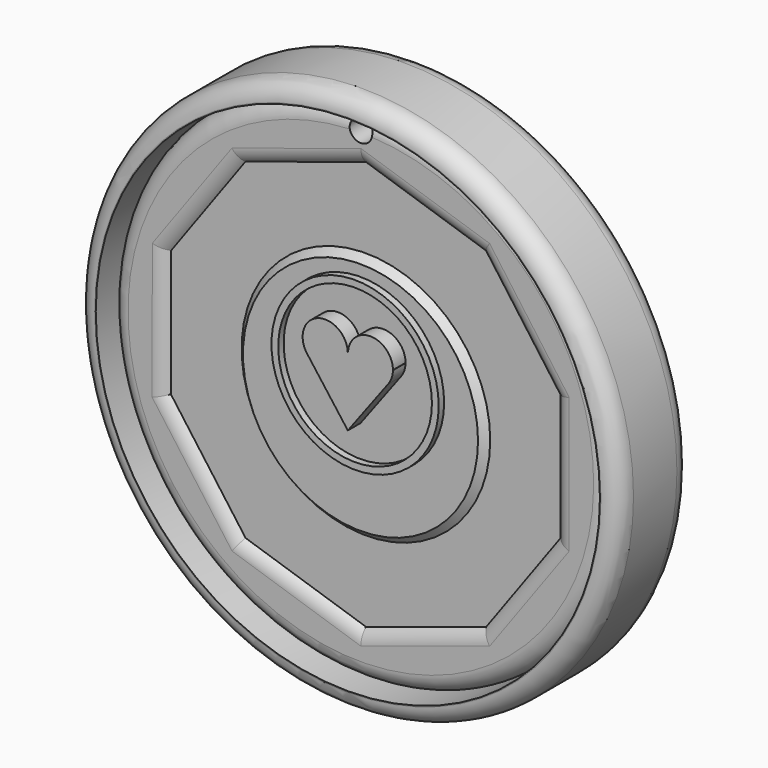
from build123d import *

# Parameters (mm, degrees)
F0_R          = 76.2
F0_R_2        = 70.8290546177
F1_DEPTH      = 25.4
F2_R          = 5.08
F4_DEPTH      = 20.828
F5_R          = 58.42
F6_DEPTH      = 19.05
F7_R          = 38.1
F8_DEPTH      = 20.955
F9_T4_DEPTH   = 54.8412301486
F9_T10_DEPTH  = 54.8210989977
F9_T16_DEPTH  = 54.8418216268
F9_T22_DEPTH  = 54.834061941
F9_T28_DEPTH  = 54.8364529893
F9_T34_DEPTH  = 54.8922066352
F9_T40_DEPTH  = 54.8735006381
F9_T46_DEPTH  = 54.8412936205
F9_T52_DEPTH  = 54.8773174101
F9_T58_DEPTH  = 54.8413615597
F9_T67_DEPTH  = 54.8412301486
F9_T71_DEPTH  = 54.8413615597
F9_T78_DEPTH  = 54.8412301486
F9_T82_DEPTH  = 54.8210989977
F9_T89_DEPTH  = 54.8210989977
F9_T93_DEPTH  = 54.8418216268
F9_T100_DEPTH = 54.8418216268
F9_T104_DEPTH = 54.834061941
F9_T111_DEPTH = 54.834061941
F9_T115_DEPTH = 54.8364529893
F9_T122_DEPTH = 54.8364529893
F9_T126_DEPTH = 54.8922066352
F9_T133_DEPTH = 54.8922066352
F9_T137_DEPTH = 54.8735006381
F9_T144_DEPTH = 54.8735006381
F9_T148_DEPTH = 54.8412936205
F9_T155_DEPTH = 54.8412936205
F9_T159_DEPTH = 54.8773174101
F9_T166_DEPTH = 54.8773174101
F9_T170_DEPTH = 54.8413615597
F12_DEPTH     = 25.4
F14_D         = 6.35
F15_R         = 23.495
F15_R_2       = 21.59
F16_DEPTH     = 22.86


# Not quite as in the source:
# - a fillet or chamfer that OpenCascade refuses, or shapes differently, is made with other operations: its cross-section is extruded or revolved along the edge and cut away or added
# - a feature names something its author has since deleted; it is built from what else it names


with BuildPart() as f1:
    # F0 (on Front) → F1 (new body)
    with BuildSketch(Plane.XZ):
        Circle(F0_R)
        Circle(F0_R_2, mode=Mode.SUBTRACT)
    extrude(amount=F1_DEPTH)

    # F2
    f2_edges = [f1.edges().sort_by_distance(p)[0] for p in [
        (76.2, -12.7, 0),
        (-76.2, 0, 0),
        (-76.2, -25.4, 0),
    ]]
    fillet(f2_edges, radius=F2_R)


with BuildPart() as f4:
    # F3 (on Front) → F4 (new body)
    with BuildSketch(Plane.XZ):
        with BuildLine():
            ThreePointArc((66.9302043248, -22.1240943887), (69.5958852645, -11.2044882855), (70.4920407102, 0))
            ThreePointArc((70.4920407102, 0), (69.6666544261, 10.7556991663), (67.2098243524, 21.2595229017))
            Line((67.2098243524, 21.2595229017), (54.6848949384, 17.7593848735))
            Line((54.6848949384, 17.7593848735), (54.6797294814, -17.7593848735))
            Line((54.6797294814, -17.7593848735), (66.9302043248, -22.1240943887))
        make_face()
        with BuildLine():
            Line((54.6848949384, 17.7593848735), (67.2098243524, 21.2595229017))
            ThreePointArc((67.2098243524, 21.2595229017), (57.3909347279, 40.9317531329), (41.9889338997, 56.6220560687))
            Line((41.9889338997, 56.6220560687), (33.8033564444, 46.5165553507))
            Line((33.8033564444, 46.5165553507), (54.6848949384, 17.7593848735))
        make_face()
        with BuildLine():
            ThreePointArc((41.8571007117, -56.719581482), (57.0778535518, -41.3672145231), (66.9302043248, -22.1240943887))
            Line((66.9302043248, -22.1240943887), (54.6797294814, -17.7593848735))
            Line((54.6797294814, -17.7593848735), (33.7952184523, -46.5151276761))
            Line((33.7952184523, -46.5151276761), (41.8571007117, -56.719581482))
        make_face()
        with BuildLine():
            Line((33.8033564444, 46.5165553507), (41.9889338997, 56.6220560687))
            ThreePointArc((41.9889338997, 56.6220560687), (22.1102184747, 66.9347894781), (0, 70.4920407102))
            Line((0, 70.4920407102), (0, 57.4872407102))
            Line((0, 57.4872407102), (33.8033564444, 46.5165553507))
        make_face()
        with BuildLine():
            ThreePointArc((0, -70.4920407102), (22.0323484517, -66.960461656), (41.8571007117, -56.719581482))
            Line((41.8571007117, -56.719581482), (33.7952184523, -46.5151276761))
            Line((33.7952184523, -46.5151276761), (0, -57.4872407102))
            Line((0, -57.4872407102), (0, -70.4920407102))
        make_face()
        with BuildLine():
            Line((0, 57.4872407102), (0, 70.4920407102))
            ThreePointArc((0, 70.4920407102), (-22.5082471688, 66.8019955755), (-42.6600170071, 56.1181855768))
            Line((-42.6600170071, 56.1181855768), (-33.8520696606, 46.5502763705))
            Line((-33.8520696606, 46.5502763705), (0, 57.4872407102))
        make_face()
        with BuildLine():
            ThreePointArc((-40.8179057709, -57.4719616158), (-21.422090766, -67.1581851355), (0, -70.4920407102))
            Line((0, -70.4920407102), (0, -57.4872407102))
            Line((0, -57.4872407102), (-33.8003104429, -46.5230722268))
            Line((-33.8003104429, -46.5230722268), (-40.8179057709, -57.4719616158))
        make_face()
        with BuildLine():
            Line((-33.8520696606, 46.5502763705), (-42.6600170071, 56.1181855768))
            ThreePointArc((-42.6600170071, 56.1181855768), (-57.0935427408, 41.3455581748), (-66.6260754104, 23.0237676955))
            Line((-66.6260754104, 23.0237676955), (-54.722988429, 17.7853191319))
            Line((-54.722988429, 17.7853191319), (-33.8520696606, 46.5502763705))
        make_face()
        with BuildLine():
            ThreePointArc((-67.6308946717, -19.8793835265), (-57.3897731413, -40.9333817596), (-40.8179057709, -57.4719616158))
            Line((-40.8179057709, -57.4719616158), (-33.8003104429, -46.5230722268))
            Line((-33.8003104429, -46.5230722268), (-54.7957226795, -17.7857782694))
            Line((-54.7957226795, -17.7857782694), (-67.6308946717, -19.8793835265))
        make_face()
        with BuildLine():
            Line((-54.722988429, 17.7853191319), (-66.6260754104, 23.0237676955))
            ThreePointArc((-66.6260754104, 23.0237676955), (-70.4727152882, 1.6505160973), (-67.6308946717, -19.8793835265))
            Line((-67.6308946717, -19.8793835265), (-54.7957226795, -17.7857782694))
            Line((-54.7957226795, -17.7857782694), (-54.722988429, 17.7853191319))
        make_face()
    extrude(amount=F4_DEPTH)

    # F5 (on Front) → F6 (join)
    with BuildSketch(Plane.XZ):
        Circle(F5_R)
    extrude(amount=F6_DEPTH)

    # F7 (on Front) → F8 (join)
    with BuildSketch(Plane.XZ):
        Circle(F7_R)
    extrude(amount=F8_DEPTH)

    # F9: fillet of radius 5.08 on 11 edges, made by hand


with BuildPart() as f9_tool2:
    # F9_s3 → F9_t4 (new body)
    with BuildSketch(Plane(origin=(-16.1166422443, 0, 22.1951571561), x_dir=(0, 1, 0), z_dir=(0.5875684882, 0, -0.8091744383))):
        with BuildLine():
            ThreePointArc((-20.828, 58.5449398441), (-20.3621391396, 56.4198233767), (-19.05, 54.6844740691))
            Line((-19.05, 54.6844740691), (-20.828, 54.6844740691))
            Line((-20.828, 54.6844740691), (-20.828, 58.5449398441))
        make_face()
    extrude(amount=F9_T4_DEPTH)

    split(bisect_by=Plane(origin=(54.6823110534, 0, -0.0079523905), x_dir=(0, 1, 0), z_dir=(-0.9999999894, 0, 0.0001454289)), keep=Keep.TOP)

    split(bisect_by=Plane(origin=(16.8792770905, 0, 52.0091681892), x_dir=(0, 1, 0), z_dir=(-0.3086939776, 0, -0.9511614102)), keep=Keep.TOP)


with BuildPart() as f4_1:
    add(f4.part)

    # F9_t1: cut F9_tool2
    add(f9_tool2.part, mode=Mode.SUBTRACT)


with BuildPart() as f9_tool8:
    # F9_s9 → F9_t10 (new body)
    with BuildSketch(Plane(origin=(0.0039874436, 0, 27.4185015995), x_dir=(0, 1, 0), z_dir=(-0.0001454289, 0, -0.9999999894))):
        with BuildLine():
            ThreePointArc((-20.828, 58.5427774067), (-20.3621391396, 56.4176609393), (-19.05, 54.6823116317))
            Line((-19.05, 54.6823116317), (-20.828, 54.6823116317))
            Line((-20.828, 54.6823116317), (-20.828, 58.5427774067))
        make_face()
    extrude(amount=F9_T10_DEPTH)

    split(bisect_by=Plane(origin=(44.2492785906, 0, 32.1308737575), x_dir=(0, 1, 0), z_dir=(-0.8091744383, 0, -0.5875684882)), keep=Keep.TOP)

    split(bisect_by=Plane(origin=(44.2416517248, 0, -32.1315039481), x_dir=(0, 1, 0), z_dir=(-0.8091207999, 0, 0.5876423497)), keep=Keep.TOP)


with BuildPart() as f4_2:
    add(f4_1.part)

    # F9_t7: cut F9_tool8
    add(f9_tool8.part, mode=Mode.SUBTRACT)


with BuildPart() as f9_tool14:
    # F9_s15 → F9_t16 (new body)
    with BuildSketch(Plane(origin=(16.1095107044, 0, 22.181076964), x_dir=(0, 1, 0), z_dir=(-0.5876423497, 0, -0.8091207999))):
        with BuildLine():
            ThreePointArc((-20.828, 58.5391388871), (-20.3621391396, 56.4140224197), (-19.05, 54.6786731121))
            Line((-19.05, 54.6786731121), (-20.828, 54.6786731121))
            Line((-20.828, 54.6786731121), (-20.828, 58.5391388871))
        make_face()
    extrude(amount=F9_T16_DEPTH)

    split(bisect_by=Plane(origin=(54.6823110534, 0, -0.0079523905), x_dir=(0, 1, 0), z_dir=(-0.9999999894, 0, 0.0001454289)), keep=Keep.TOP)

    split(bisect_by=Plane(origin=(16.8843448329, 0, -52.0054906728), x_dir=(0, 1, 0), z_dir=(-0.3087975758, 0, 0.9511277817)), keep=Keep.TOP)


with BuildPart() as f4_3:
    add(f4_2.part)

    # F9_t13: cut F9_tool14
    add(f9_tool14.part, mode=Mode.SUBTRACT)


with BuildPart() as f9_tool20:
    # F9_s21 → F9_t22 (new body)
    with BuildSketch(Plane(origin=(26.0903642421, 0, 8.4706191785), x_dir=(0, 1, 0), z_dir=(-0.9511277817, 0, -0.3087975758))):
        with BuildLine():
            ThreePointArc((-20.828, 58.5381775099), (-20.3621391396, 56.4130610425), (-19.05, 54.6777117348))
            Line((-19.05, 54.6777117348), (-20.828, 54.6777117348))
            Line((-20.828, 54.6777117348), (-20.828, 58.5381775099))
        make_face()
    extrude(amount=F9_T22_DEPTH)

    split(bisect_by=Plane(origin=(44.2416517248, 0, -32.1315039481), x_dir=(0, 1, 0), z_dir=(-0.8091207999, 0, 0.5876423497)), keep=Keep.TOP)

    split(bisect_by=Plane(origin=(-16.8723907072, 0, -52.0141627411), x_dir=(0, 1, 0), z_dir=(0.3085532219, 0, 0.9512070801)), keep=Keep.TOP)


with BuildPart() as f4_4:
    add(f4_3.part)

    # F9_t19: cut F9_tool20
    add(f9_tool20.part, mode=Mode.SUBTRACT)


with BuildPart() as f9_tool26:
    # F9_s27 → F9_t28 (new body)
    with BuildSketch(Plane(origin=(26.0526466514, 0, -8.4509758515), x_dir=(0, 1, 0), z_dir=(-0.9512070801, 0, 0.3085532219))):
        with BuildLine():
            ThreePointArc((-20.828, 58.5427361543), (-20.3621391396, 56.4176196869), (-19.05, 54.6822703793))
            Line((-19.05, 54.6822703793), (-20.828, 54.6822703793))
            Line((-20.828, 54.6822703793), (-20.828, 58.5427361543))
        make_face()
    extrude(amount=F9_T28_DEPTH)

    split(bisect_by=Plane(origin=(16.8843448329, 0, -52.0054906728), x_dir=(0, 1, 0), z_dir=(-0.3087975758, 0, 0.9511277817)), keep=Keep.TOP)

    split(bisect_by=Plane(origin=(-44.1981655034, 0, -32.2910955438), x_dir=(0, 1, 0), z_dir=(0.8074569447, 0, 0.589926506)), keep=Keep.TOP)


with BuildPart() as f4_5:
    add(f4_4.part)

    # F9_t25: cut F9_tool26
    add(f9_tool26.part, mode=Mode.SUBTRACT)


with BuildPart() as f9_tool32:
    # F9_s33 → F9_t34 (new body)
    with BuildSketch(Plane(origin=(16.0913327762, 0, -22.0248764322), x_dir=(0, 1, 0), z_dir=(-0.589926506, 0, 0.8074569447))):
        with BuildLine():
            ThreePointArc((-20.828, 58.5979546221), (-20.3621391396, 56.4728381547), (-19.05, 54.7374888471))
            Line((-19.05, 54.7374888471), (-20.828, 54.7374888471))
            Line((-20.828, 54.7374888471), (-20.828, 58.5979546221))
        make_face()
    extrude(amount=F9_T34_DEPTH)

    split(bisect_by=Plane(origin=(-16.8723907072, 0, -52.0141627411), x_dir=(0, 1, 0), z_dir=(0.3085532219, 0, 0.9512070801)), keep=Keep.TOP)

    split(bisect_by=Plane(origin=(-54.7591261352, 0, 0.1119691067), x_dir=(0, 1, 0), z_dir=(0.9999979095, 0, -0.0020447527)), keep=Keep.TOP)


with BuildPart() as f4_6:
    add(f4_5.part)

    # F9_t31: cut F9_tool32
    add(f9_tool32.part, mode=Mode.SUBTRACT)


with BuildPart() as f9_tool38:
    # F9_s39 → F9_t40 (new body)
    with BuildSketch(Plane(origin=(-0.0563307891, 0, -27.5488916378), x_dir=(0, 1, 0), z_dir=(0.0020447527, 0, 0.9999979095))):
        with BuildLine():
            ThreePointArc((-20.828, 58.6197063849), (-20.3621391396, 56.4945899175), (-19.05, 54.7592406099))
            Line((-19.05, 54.7592406099), (-20.828, 54.7592406099))
            Line((-20.828, 54.7592406099), (-20.828, 58.6197063849))
        make_face()
    extrude(amount=F9_T40_DEPTH)

    split(bisect_by=Plane(origin=(-44.1981655034, 0, -32.2910955438), x_dir=(0, 1, 0), z_dir=(0.8074569447, 0, 0.589926506)), keep=Keep.TOP)

    split(bisect_by=Plane(origin=(-44.3037877316, 0, 32.1453895171), x_dir=(0, 1, 0), z_dir=(0.8093920981, 0, -0.5872686196)), keep=Keep.TOP)


with BuildPart() as f4_7:
    add(f4_6.part)

    # F9_t37: cut F9_tool38
    add(f9_tool38.part, mode=Mode.SUBTRACT)


with BuildPart() as f9_tool44:
    # F9_s45 → F9_t46 (new body)
    with BuildSketch(Plane(origin=(-16.0870267142, 0, -22.1716466182), x_dir=(0, 1, 0), z_dir=(0.5872686196, 0, 0.8093920981))):
        with BuildLine():
            ThreePointArc((-20.828, 58.5975800082), (-20.3621391396, 56.4724635408), (-19.05, 54.7371142332))
            Line((-19.05, 54.7371142332), (-20.828, 54.7371142332))
            Line((-20.828, 54.7371142332), (-20.828, 58.5975800082))
        make_face()
    extrude(amount=F9_T46_DEPTH)

    split(bisect_by=Plane(origin=(-54.7591261352, 0, 0.1119691067), x_dir=(0, 1, 0), z_dir=(0.9999979095, 0, -0.0020447527)), keep=Keep.TOP)

    split(bisect_by=Plane(origin=(-16.8175972659, 0, 52.0537926693), x_dir=(0, 1, 0), z_dir=(0.3074340932, 0, -0.9515693765)), keep=Keep.TOP)


with BuildPart() as f4_8:
    add(f4_7.part)

    # F9_t43: cut F9_tool44
    add(f9_tool44.part, mode=Mode.SUBTRACT)


with BuildPart() as f9_tool50:
    # F9_s51 → F9_t52 (new body)
    with BuildSketch(Plane(origin=(-26.2182249213, 0, -8.4706132857), x_dir=(0, 1, 0), z_dir=(0.9515693765, 0, 0.3074340932))):
        with BuildLine():
            ThreePointArc((-20.828, 58.5635635763), (-20.3621391396, 56.4384471089), (-19.05, 54.7030978013))
            Line((-19.05, 54.7030978013), (-20.828, 54.7030978013))
            Line((-20.828, 54.7030978013), (-20.828, 58.5635635763))
        make_face()
    extrude(amount=F9_T52_DEPTH)

    split(bisect_by=Plane(origin=(-44.3037877316, 0, 32.1453895171), x_dir=(0, 1, 0), z_dir=(0.8093920981, 0, -0.5872686196)), keep=Keep.TOP)

    split(bisect_by=Plane(origin=(16.8792770905, 0, 52.0091681892), x_dir=(0, 1, 0), z_dir=(-0.3086939776, 0, -0.9511614102)), keep=Keep.TOP)


with BuildPart() as f4_9:
    add(f4_8.part)

    # F9_t49: cut F9_tool50
    add(f9_tool50.part, mode=Mode.SUBTRACT)


with BuildPart() as f9_tool56:
    # F9_s57 → F9_t58 (new body)
    with BuildSketch(Plane(origin=(-26.0590922666, 0, 8.4573288597), x_dir=(0, 1, 0), z_dir=(0.9511614102, 0, -0.3086939776))):
        with BuildLine():
            ThreePointArc((-20.828, 58.5401107156), (-20.3621391396, 56.4149942482), (-19.05, 54.6796449406))
            Line((-19.05, 54.6796449406), (-20.828, 54.6796449406))
            Line((-20.828, 54.6796449406), (-20.828, 58.5401107156))
        make_face()
    extrude(amount=F9_T58_DEPTH)

    split(bisect_by=Plane(origin=(44.2492785906, 0, 32.1308737575), x_dir=(0, 1, 0), z_dir=(-0.8091744383, 0, -0.5875684882)), keep=Keep.TOP)

    split(bisect_by=Plane(origin=(-16.8175972659, 0, 52.0537926693), x_dir=(0, 1, 0), z_dir=(0.3074340932, 0, -0.9515693765)), keep=Keep.TOP)


with BuildPart() as f4_10:
    add(f4_9.part)

    # F9_t55: cut F9_tool56
    add(f9_tool56.part, mode=Mode.SUBTRACT)

    # F9_s61 → F9_t62 (revolve, cut)
    with BuildSketch(Plane(origin=(0, 0, 0), x_dir=(0, 1, 0), z_dir=(0.3266151393, 0, 0.9451574212))):
        with BuildLine():
            ThreePointArc((-15.748, 70.4920407102), (-19.3401024484, 69.0041431586), (-20.828, 65.4120407102))
            Line((-20.828, 65.4120407102), (-20.828, 70.4920407102))
            Line((-20.828, 70.4920407102), (-15.748, 70.4920407102))
        make_face()
    revolve(axis=Axis((0, -20.828, 0), (0, -1, 0)), mode=Mode.SUBTRACT)


with BuildPart() as f9_tool65:
    # F9_s66 → F9_t67 (new body)
    with BuildSketch(Plane(origin=(-16.1166422443, 0, 22.1951571561), x_dir=(0, 1, 0), z_dir=(0.5875684882, 0, -0.8091744383))):
        with BuildLine():
            ThreePointArc((-20.828, 58.5449398441), (-20.3621391396, 56.4198233767), (-19.05, 54.6844740691))
            Line((-19.05, 54.6844740691), (-20.828, 54.6844740691))
            Line((-20.828, 54.6844740691), (-20.828, 58.5449398441))
        make_face()
    extrude(amount=F9_T67_DEPTH)

    split(bisect_by=Plane(origin=(16.8792770905, 0, 52.0091681892), x_dir=(0, 1, 0), z_dir=(0.3086939776, 0, 0.9511614102)), keep=Keep.TOP)


with BuildPart() as f9_tool69:
    # F9_s70 → F9_t71 (new body)
    with BuildSketch(Plane(origin=(-26.0590922666, 0, 8.4573288597), x_dir=(0, 1, 0), z_dir=(0.9511614102, 0, -0.3086939776))):
        with BuildLine():
            ThreePointArc((-20.828, 58.5401107156), (-20.3621391396, 56.4149942482), (-19.05, 54.6796449406))
            Line((-19.05, 54.6796449406), (-20.828, 54.6796449406))
            Line((-20.828, 54.6796449406), (-20.828, 58.5401107156))
        make_face()
    extrude(amount=F9_T71_DEPTH)

    split(bisect_by=Plane(origin=(44.2492785906, 0, 32.1308737575), x_dir=(0, 1, 0), z_dir=(0.8091744383, 0, 0.5875684882)), keep=Keep.TOP)


with BuildPart() as f9_tool65_1:
    add(f9_tool65.part)

    # F9_t73: intersect F9_tool69
    add(f9_tool69.part, mode=Mode.INTERSECT)


with BuildPart() as f4_11:
    add(f4_10.part)

    # F9_t63: cut F9_tool65
    add(f9_tool65_1.part, mode=Mode.SUBTRACT)


with BuildPart() as f9_tool76:
    # F9_s77 → F9_t78 (new body)
    with BuildSketch(Plane(origin=(-16.1166422443, 0, 22.1951571561), x_dir=(0, 1, 0), z_dir=(0.5875684882, 0, -0.8091744383))):
        with BuildLine():
            ThreePointArc((-20.828, 58.5449398441), (-20.3621391396, 56.4198233767), (-19.05, 54.6844740691))
            Line((-19.05, 54.6844740691), (-20.828, 54.6844740691))
            Line((-20.828, 54.6844740691), (-20.828, 58.5449398441))
        make_face()
    extrude(amount=F9_T78_DEPTH)

    split(bisect_by=Plane(origin=(54.6823110534, 0, -0.0079523905), x_dir=(0, 1, 0), z_dir=(0.9999999894, 0, -0.0001454289)), keep=Keep.TOP)


with BuildPart() as f9_tool80:
    # F9_s81 → F9_t82 (new body)
    with BuildSketch(Plane(origin=(0.0039874436, 0, 27.4185015995), x_dir=(0, 1, 0), z_dir=(-0.0001454289, 0, -0.9999999894))):
        with BuildLine():
            ThreePointArc((-20.828, 58.5427774067), (-20.3621391396, 56.4176609393), (-19.05, 54.6823116317))
            Line((-19.05, 54.6823116317), (-20.828, 54.6823116317))
            Line((-20.828, 54.6823116317), (-20.828, 58.5427774067))
        make_face()
    extrude(amount=F9_T82_DEPTH)

    split(bisect_by=Plane(origin=(44.2492785906, 0, 32.1308737575), x_dir=(0, 1, 0), z_dir=(0.8091744383, 0, 0.5875684882)), keep=Keep.TOP)


with BuildPart() as f9_tool76_1:
    add(f9_tool76.part)

    # F9_t84: intersect F9_tool80
    add(f9_tool80.part, mode=Mode.INTERSECT)


with BuildPart() as f4_12:
    add(f4_11.part)

    # F9_t74: cut F9_tool76
    add(f9_tool76_1.part, mode=Mode.SUBTRACT)


with BuildPart() as f9_tool87:
    # F9_s88 → F9_t89 (new body)
    with BuildSketch(Plane(origin=(0.0039874436, 0, 27.4185015995), x_dir=(0, 1, 0), z_dir=(-0.0001454289, 0, -0.9999999894))):
        with BuildLine():
            ThreePointArc((-20.828, 58.5427774067), (-20.3621391396, 56.4176609393), (-19.05, 54.6823116317))
            Line((-19.05, 54.6823116317), (-20.828, 54.6823116317))
            Line((-20.828, 54.6823116317), (-20.828, 58.5427774067))
        make_face()
    extrude(amount=F9_T89_DEPTH)

    split(bisect_by=Plane(origin=(44.2416517248, 0, -32.1315039481), x_dir=(0, 1, 0), z_dir=(0.8091207999, 0, -0.5876423497)), keep=Keep.TOP)


with BuildPart() as f9_tool91:
    # F9_s92 → F9_t93 (new body)
    with BuildSketch(Plane(origin=(16.1095107044, 0, 22.181076964), x_dir=(0, 1, 0), z_dir=(-0.5876423497, 0, -0.8091207999))):
        with BuildLine():
            ThreePointArc((-20.828, 58.5391388871), (-20.3621391396, 56.4140224197), (-19.05, 54.6786731121))
            Line((-19.05, 54.6786731121), (-20.828, 54.6786731121))
            Line((-20.828, 54.6786731121), (-20.828, 58.5391388871))
        make_face()
    extrude(amount=F9_T93_DEPTH)

    split(bisect_by=Plane(origin=(54.6823110534, 0, -0.0079523905), x_dir=(0, 1, 0), z_dir=(0.9999999894, 0, -0.0001454289)), keep=Keep.TOP)


with BuildPart() as f9_tool87_1:
    add(f9_tool87.part)

    # F9_t95: intersect F9_tool91
    add(f9_tool91.part, mode=Mode.INTERSECT)


with BuildPart() as f4_13:
    add(f4_12.part)

    # F9_t85: cut F9_tool87
    add(f9_tool87_1.part, mode=Mode.SUBTRACT)


with BuildPart() as f9_tool98:
    # F9_s99 → F9_t100 (new body)
    with BuildSketch(Plane(origin=(16.1095107044, 0, 22.181076964), x_dir=(0, 1, 0), z_dir=(-0.5876423497, 0, -0.8091207999))):
        with BuildLine():
            ThreePointArc((-20.828, 58.5391388871), (-20.3621391396, 56.4140224197), (-19.05, 54.6786731121))
            Line((-19.05, 54.6786731121), (-20.828, 54.6786731121))
            Line((-20.828, 54.6786731121), (-20.828, 58.5391388871))
        make_face()
    extrude(amount=F9_T100_DEPTH)

    split(bisect_by=Plane(origin=(16.8843448329, 0, -52.0054906728), x_dir=(0, 1, 0), z_dir=(0.3087975758, 0, -0.9511277817)), keep=Keep.TOP)


with BuildPart() as f9_tool102:
    # F9_s103 → F9_t104 (new body)
    with BuildSketch(Plane(origin=(26.0903642421, 0, 8.4706191785), x_dir=(0, 1, 0), z_dir=(-0.9511277817, 0, -0.3087975758))):
        with BuildLine():
            ThreePointArc((-20.828, 58.5381775099), (-20.3621391396, 56.4130610425), (-19.05, 54.6777117348))
            Line((-19.05, 54.6777117348), (-20.828, 54.6777117348))
            Line((-20.828, 54.6777117348), (-20.828, 58.5381775099))
        make_face()
    extrude(amount=F9_T104_DEPTH)

    split(bisect_by=Plane(origin=(44.2416517248, 0, -32.1315039481), x_dir=(0, 1, 0), z_dir=(0.8091207999, 0, -0.5876423497)), keep=Keep.TOP)


with BuildPart() as f9_tool98_1:
    add(f9_tool98.part)

    # F9_t106: intersect F9_tool102
    add(f9_tool102.part, mode=Mode.INTERSECT)


with BuildPart() as f4_14:
    add(f4_13.part)

    # F9_t96: cut F9_tool98
    add(f9_tool98_1.part, mode=Mode.SUBTRACT)


with BuildPart() as f9_tool109:
    # F9_s110 → F9_t111 (new body)
    with BuildSketch(Plane(origin=(26.0903642421, 0, 8.4706191785), x_dir=(0, 1, 0), z_dir=(-0.9511277817, 0, -0.3087975758))):
        with BuildLine():
            ThreePointArc((-20.828, 58.5381775099), (-20.3621391396, 56.4130610425), (-19.05, 54.6777117348))
            Line((-19.05, 54.6777117348), (-20.828, 54.6777117348))
            Line((-20.828, 54.6777117348), (-20.828, 58.5381775099))
        make_face()
    extrude(amount=F9_T111_DEPTH)

    split(bisect_by=Plane(origin=(-16.8723907072, 0, -52.0141627411), x_dir=(0, 1, 0), z_dir=(-0.3085532219, 0, -0.9512070801)), keep=Keep.TOP)


with BuildPart() as f9_tool113:
    # F9_s114 → F9_t115 (new body)
    with BuildSketch(Plane(origin=(26.0526466514, 0, -8.4509758515), x_dir=(0, 1, 0), z_dir=(-0.9512070801, 0, 0.3085532219))):
        with BuildLine():
            ThreePointArc((-20.828, 58.5427361543), (-20.3621391396, 56.4176196869), (-19.05, 54.6822703793))
            Line((-19.05, 54.6822703793), (-20.828, 54.6822703793))
            Line((-20.828, 54.6822703793), (-20.828, 58.5427361543))
        make_face()
    extrude(amount=F9_T115_DEPTH)

    split(bisect_by=Plane(origin=(16.8843448329, 0, -52.0054906728), x_dir=(0, 1, 0), z_dir=(0.3087975758, 0, -0.9511277817)), keep=Keep.TOP)


with BuildPart() as f9_tool109_1:
    add(f9_tool109.part)

    # F9_t117: intersect F9_tool113
    add(f9_tool113.part, mode=Mode.INTERSECT)


with BuildPart() as f4_15:
    add(f4_14.part)

    # F9_t107: cut F9_tool109
    add(f9_tool109_1.part, mode=Mode.SUBTRACT)


with BuildPart() as f9_tool120:
    # F9_s121 → F9_t122 (new body)
    with BuildSketch(Plane(origin=(26.0526466514, 0, -8.4509758515), x_dir=(0, 1, 0), z_dir=(-0.9512070801, 0, 0.3085532219))):
        with BuildLine():
            ThreePointArc((-20.828, 58.5427361543), (-20.3621391396, 56.4176196869), (-19.05, 54.6822703793))
            Line((-19.05, 54.6822703793), (-20.828, 54.6822703793))
            Line((-20.828, 54.6822703793), (-20.828, 58.5427361543))
        make_face()
    extrude(amount=F9_T122_DEPTH)

    split(bisect_by=Plane(origin=(-44.1981655034, 0, -32.2910955438), x_dir=(0, 1, 0), z_dir=(-0.8074569447, 0, -0.589926506)), keep=Keep.TOP)


with BuildPart() as f9_tool124:
    # F9_s125 → F9_t126 (new body)
    with BuildSketch(Plane(origin=(16.0913327762, 0, -22.0248764322), x_dir=(0, 1, 0), z_dir=(-0.589926506, 0, 0.8074569447))):
        with BuildLine():
            ThreePointArc((-20.828, 58.5979546221), (-20.3621391396, 56.4728381547), (-19.05, 54.7374888471))
            Line((-19.05, 54.7374888471), (-20.828, 54.7374888471))
            Line((-20.828, 54.7374888471), (-20.828, 58.5979546221))
        make_face()
    extrude(amount=F9_T126_DEPTH)

    split(bisect_by=Plane(origin=(-16.8723907072, 0, -52.0141627411), x_dir=(0, 1, 0), z_dir=(-0.3085532219, 0, -0.9512070801)), keep=Keep.TOP)


with BuildPart() as f9_tool120_1:
    add(f9_tool120.part)

    # F9_t128: intersect F9_tool124
    add(f9_tool124.part, mode=Mode.INTERSECT)


with BuildPart() as f4_16:
    add(f4_15.part)

    # F9_t118: cut F9_tool120
    add(f9_tool120_1.part, mode=Mode.SUBTRACT)


with BuildPart() as f9_tool131:
    # F9_s132 → F9_t133 (new body)
    with BuildSketch(Plane(origin=(16.0913327762, 0, -22.0248764322), x_dir=(0, 1, 0), z_dir=(-0.589926506, 0, 0.8074569447))):
        with BuildLine():
            ThreePointArc((-20.828, 58.5979546221), (-20.3621391396, 56.4728381547), (-19.05, 54.7374888471))
            Line((-19.05, 54.7374888471), (-20.828, 54.7374888471))
            Line((-20.828, 54.7374888471), (-20.828, 58.5979546221))
        make_face()
    extrude(amount=F9_T133_DEPTH)

    split(bisect_by=Plane(origin=(-54.7591261352, 0, 0.1119691067), x_dir=(0, 1, 0), z_dir=(-0.9999979095, 0, 0.0020447527)), keep=Keep.TOP)


with BuildPart() as f9_tool135:
    # F9_s136 → F9_t137 (new body)
    with BuildSketch(Plane(origin=(-0.0563307891, 0, -27.5488916378), x_dir=(0, 1, 0), z_dir=(0.0020447527, 0, 0.9999979095))):
        with BuildLine():
            ThreePointArc((-20.828, 58.6197063849), (-20.3621391396, 56.4945899175), (-19.05, 54.7592406099))
            Line((-19.05, 54.7592406099), (-20.828, 54.7592406099))
            Line((-20.828, 54.7592406099), (-20.828, 58.6197063849))
        make_face()
    extrude(amount=F9_T137_DEPTH)

    split(bisect_by=Plane(origin=(-44.1981655034, 0, -32.2910955438), x_dir=(0, 1, 0), z_dir=(-0.8074569447, 0, -0.589926506)), keep=Keep.TOP)


with BuildPart() as f9_tool131_1:
    add(f9_tool131.part)

    # F9_t139: intersect F9_tool135
    add(f9_tool135.part, mode=Mode.INTERSECT)


with BuildPart() as f4_17:
    add(f4_16.part)

    # F9_t129: cut F9_tool131
    add(f9_tool131_1.part, mode=Mode.SUBTRACT)


with BuildPart() as f9_tool142:
    # F9_s143 → F9_t144 (new body)
    with BuildSketch(Plane(origin=(-0.0563307891, 0, -27.5488916378), x_dir=(0, 1, 0), z_dir=(0.0020447527, 0, 0.9999979095))):
        with BuildLine():
            ThreePointArc((-20.828, 58.6197063849), (-20.3621391396, 56.4945899175), (-19.05, 54.7592406099))
            Line((-19.05, 54.7592406099), (-20.828, 54.7592406099))
            Line((-20.828, 54.7592406099), (-20.828, 58.6197063849))
        make_face()
    extrude(amount=F9_T144_DEPTH)

    split(bisect_by=Plane(origin=(-44.3037877316, 0, 32.1453895171), x_dir=(0, 1, 0), z_dir=(-0.8093920981, 0, 0.5872686196)), keep=Keep.TOP)


with BuildPart() as f9_tool146:
    # F9_s147 → F9_t148 (new body)
    with BuildSketch(Plane(origin=(-16.0870267142, 0, -22.1716466182), x_dir=(0, 1, 0), z_dir=(0.5872686196, 0, 0.8093920981))):
        with BuildLine():
            ThreePointArc((-20.828, 58.5975800082), (-20.3621391396, 56.4724635408), (-19.05, 54.7371142332))
            Line((-19.05, 54.7371142332), (-20.828, 54.7371142332))
            Line((-20.828, 54.7371142332), (-20.828, 58.5975800082))
        make_face()
    extrude(amount=F9_T148_DEPTH)

    split(bisect_by=Plane(origin=(-54.7591261352, 0, 0.1119691067), x_dir=(0, 1, 0), z_dir=(-0.9999979095, 0, 0.0020447527)), keep=Keep.TOP)


with BuildPart() as f9_tool142_1:
    add(f9_tool142.part)

    # F9_t150: intersect F9_tool146
    add(f9_tool146.part, mode=Mode.INTERSECT)


with BuildPart() as f4_18:
    add(f4_17.part)

    # F9_t140: cut F9_tool142
    add(f9_tool142_1.part, mode=Mode.SUBTRACT)


with BuildPart() as f9_tool153:
    # F9_s154 → F9_t155 (new body)
    with BuildSketch(Plane(origin=(-16.0870267142, 0, -22.1716466182), x_dir=(0, 1, 0), z_dir=(0.5872686196, 0, 0.8093920981))):
        with BuildLine():
            ThreePointArc((-20.828, 58.5975800082), (-20.3621391396, 56.4724635408), (-19.05, 54.7371142332))
            Line((-19.05, 54.7371142332), (-20.828, 54.7371142332))
            Line((-20.828, 54.7371142332), (-20.828, 58.5975800082))
        make_face()
    extrude(amount=F9_T155_DEPTH)

    split(bisect_by=Plane(origin=(-16.8175972659, 0, 52.0537926693), x_dir=(0, 1, 0), z_dir=(-0.3074340932, 0, 0.9515693765)), keep=Keep.TOP)


with BuildPart() as f9_tool157:
    # F9_s158 → F9_t159 (new body)
    with BuildSketch(Plane(origin=(-26.2182249213, 0, -8.4706132857), x_dir=(0, 1, 0), z_dir=(0.9515693765, 0, 0.3074340932))):
        with BuildLine():
            ThreePointArc((-20.828, 58.5635635763), (-20.3621391396, 56.4384471089), (-19.05, 54.7030978013))
            Line((-19.05, 54.7030978013), (-20.828, 54.7030978013))
            Line((-20.828, 54.7030978013), (-20.828, 58.5635635763))
        make_face()
    extrude(amount=F9_T159_DEPTH)

    split(bisect_by=Plane(origin=(-44.3037877316, 0, 32.1453895171), x_dir=(0, 1, 0), z_dir=(-0.8093920981, 0, 0.5872686196)), keep=Keep.TOP)


with BuildPart() as f9_tool153_1:
    add(f9_tool153.part)

    # F9_t161: intersect F9_tool157
    add(f9_tool157.part, mode=Mode.INTERSECT)


with BuildPart() as f4_19:
    add(f4_18.part)

    # F9_t151: cut F9_tool153
    add(f9_tool153_1.part, mode=Mode.SUBTRACT)


with BuildPart() as f9_tool164:
    # F9_s165 → F9_t166 (new body)
    with BuildSketch(Plane(origin=(-26.2182249213, 0, -8.4706132857), x_dir=(0, 1, 0), z_dir=(0.9515693765, 0, 0.3074340932))):
        with BuildLine():
            ThreePointArc((-20.828, 58.5635635763), (-20.3621391396, 56.4384471089), (-19.05, 54.7030978013))
            Line((-19.05, 54.7030978013), (-20.828, 54.7030978013))
            Line((-20.828, 54.7030978013), (-20.828, 58.5635635763))
        make_face()
    extrude(amount=F9_T166_DEPTH)

    split(bisect_by=Plane(origin=(16.8792770905, 0, 52.0091681892), x_dir=(0, 1, 0), z_dir=(0.3086939776, 0, 0.9511614102)), keep=Keep.TOP)


with BuildPart() as f9_tool168:
    # F9_s169 → F9_t170 (new body)
    with BuildSketch(Plane(origin=(-26.0590922666, 0, 8.4573288597), x_dir=(0, 1, 0), z_dir=(0.9511614102, 0, -0.3086939776))):
        with BuildLine():
            ThreePointArc((-20.828, 58.5401107156), (-20.3621391396, 56.4149942482), (-19.05, 54.6796449406))
            Line((-19.05, 54.6796449406), (-20.828, 54.6796449406))
            Line((-20.828, 54.6796449406), (-20.828, 58.5401107156))
        make_face()
    extrude(amount=F9_T170_DEPTH)

    split(bisect_by=Plane(origin=(-16.8175972659, 0, 52.0537926693), x_dir=(0, 1, 0), z_dir=(-0.3074340932, 0, 0.9515693765)), keep=Keep.TOP)


with BuildPart() as f9_tool164_1:
    add(f9_tool164.part)

    # F9_t172: intersect F9_tool168
    add(f9_tool168.part, mode=Mode.INTERSECT)


with BuildPart() as f4_20:
    add(f4_19.part)

    # F9_t162: cut F9_tool164
    add(f9_tool164_1.part, mode=Mode.SUBTRACT)

    # F10: chamfer of 5.08 on 1 edges, made by hand


with BuildPart() as f10_tool2:
    # F10_s3 → F10_t4 (revolve)
    with BuildSketch(Plane.XY):
        Polygon((38.1, -15.875), (33.02, -20.955), (38.1, -20.955), align=None)
    revolve(axis=Axis((0, -20.955, 0), (0, -1, 0)))

    split(bisect_by=Plane.XZ.offset(19.05), keep=Keep.TOP)


with BuildPart() as f4_21:
    add(f4_20.part)

    # F10_t1: cut F10_tool2
    add(f10_tool2.part, mode=Mode.SUBTRACT)

    # F11 (on Front) → F12 (join)
    with BuildSketch(Plane.XZ):
        with BuildLine():
            Line((0.0390368972, 12.7), (0, 12.7))
            Line((0, 12.7), (0, 0))
            Line((0, 0), (0, -6.35))
            Line((0, -6.35), (8.831620092, 6.8974301379))
            ThreePointArc((8.831620092, 6.8974301379), (2.873878422, 7.4326634757), (0.0390368972, 12.7))
        make_face()
        with BuildLine():
            ThreePointArc((-8.7923076923, 6.8384615385), (-2.827653754, 7.416480631), (0, 12.7))
            Line((0, 12.7), (-6.35, 12.7))
            Line((-6.35, 12.7), (-12.7, 12.7))
            Line((-12.7, 12.7), (-8.7923076923, 6.8384615385))
        make_face()
        with BuildLine():
            Line((-6.35, 12.7), (0, 12.7))
            ThreePointArc((0, 12.7), (-6.35, 19.05), (-12.7, 12.7))
            Line((-12.7, 12.7), (-6.35, 12.7))
        make_face()
        with BuildLine():
            Line((0, 0), (0, 12.7))
            ThreePointArc((0, 12.7), (-2.827653754, 7.416480631), (-8.7923076923, 6.8384615385))
            Line((-8.7923076923, 6.8384615385), (0, -6.35))
            Line((0, -6.35), (0, 0))
        make_face()
        with BuildLine():
            ThreePointArc((12.6609631028, 12.7), (6.35, 19.0109631028), (0.0390368972, 12.7))
            Line((0.0390368972, 12.7), (6.35, 12.7))
            Line((6.35, 12.7), (12.6609631028, 12.7))
        make_face()
        with BuildLine():
            Line((6.35, 12.7), (0.0390368972, 12.7))
            ThreePointArc((0.0390368972, 12.7), (2.873878422, 7.4326634757), (8.831620092, 6.8974301379))
            Line((8.831620092, 6.8974301379), (12.6606876004, 12.6410314005))
            ThreePointArc((12.6606876004, 12.6410314005), (12.6608942268, 12.6705153785), (12.6609631028, 12.7))
            Line((12.6609631028, 12.7), (6.35, 12.7))
        make_face()
        with BuildLine():
            Line((-8.7923076923, 6.8384615385), (-12.7, 12.7))
            ThreePointArc((-12.7, 12.7), (-12.3429244384, 10.6006294573), (-11.3118561652, 8.7373640848))
            ThreePointArc((-11.3118561652, 8.7373640848), (-10.1718932909, 7.6289417601), (-8.7923076923, 6.8384615385))
        make_face()
        with BuildLine():
            Line((0, -6.35), (-8.7923076923, 6.8384615385))
            ThreePointArc((-8.7923076923, 6.8384615385), (-10.1718932909, 7.6289417601), (-11.3118561652, 8.7373640848))
            Line((-11.3118561652, 8.7373640848), (0, -6.35))
        make_face()
        with BuildLine():
            Line((8.831620092, 6.8974301379), (0, -6.35))
            Line((0, -6.35), (11.2769219917, 8.7561826902))
            ThreePointArc((11.2769219917, 8.7561826902), (10.1690789746, 7.6757696041), (8.831620092, 6.8974301379))
        make_face()
        with BuildLine():
            Line((12.7, 12.7), (12.6609631028, 12.7))
            ThreePointArc((12.6609631028, 12.7), (12.6608942268, 12.6705153785), (12.6606876004, 12.6410314005))
            Line((12.6606876004, 12.6410314005), (12.7, 12.7))
        make_face()
        with BuildLine():
            Line((12.6606876004, 12.6410314005), (8.831620092, 6.8974301379))
            ThreePointArc((8.831620092, 6.8974301379), (10.1690789746, 7.6757696041), (11.2769219917, 8.7561826902))
            ThreePointArc((11.2769219917, 8.7561826902), (12.2950802948, 10.5823891827), (12.6606876004, 12.6410314005))
        make_face()
    extrude(amount=F12_DEPTH)

    # F14 (through all)
    with Locations(Plane(origin=(0, 0, 0), x_dir=(1, 0, 0), z_dir=(0, 1, 0))):
        with Locations((0, -66.04)):
            Hole(F14_D / 2)

    # F15 (on Front) → F16 (join)
    with BuildSketch(Plane.XZ):
        with Locations((0, 6.35)):
            Circle(F15_R)
        with Locations((0, 6.35)):
            Circle(F15_R_2, mode=Mode.SUBTRACT)
    extrude(amount=F16_DEPTH)


solid = Compound([f1.part, f4_21.part])
